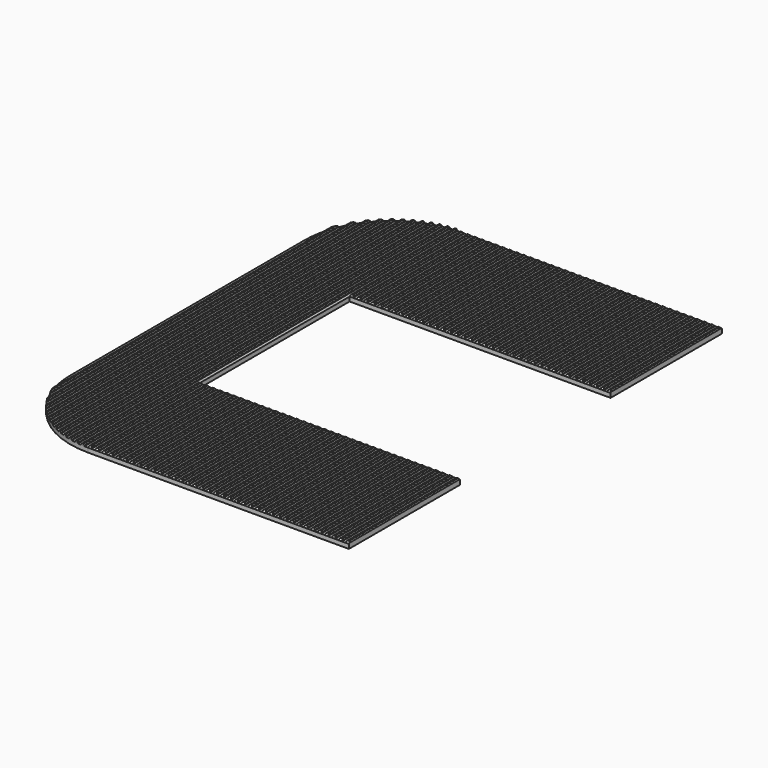
from build123d import *

# Parameters (mm, degrees)
F1_DEPTH = 2.5
F2_R     = 50
F3_W     = 2
F3_H     = 80
F4_DEPTH = 1
F5_SIZE  = 1
F6_SIZE  = 0.6


with BuildPart() as f1:
    # F0 (on Top) → F1 (new body)
    with BuildSketch(Plane.XY):
        Polygon((0, 134), (-200, 134), (-200, -134), (0, -134), (0, -54), (-150, -54), (-150, 54), (0, 54), align=None)
    extrude(amount=F1_DEPTH)

    # F2
    f2_edges = [f1.edges().sort_by_distance(p)[0] for p in [
        (-200, -134, 1.25),
        (-200, 134, 1.25),
    ]]
    fillet(f2_edges, radius=F2_R)

    # F3 (on face) → F4 (join)
    with BuildSketch(Plane.XY.offset(2.5)):
        with BuildLine():
            Line((-196, -103.5959179423), (-196, 103.5959179423))
            ThreePointArc((-196, 103.5959179423), (-197.0832090496, 100.8276981669), (-198, 98))
            Line((-198, 98), (-198, -98))
            ThreePointArc((-198, -98), (-197.0832090496, -100.8276981669), (-196, -103.5959179423))
        make_face()
        with BuildLine():
            Line((-192, -111.1293199325), (-192, 111.1293199325))
            ThreePointArc((-192, 111.1293199325), (-193.0332101351, 109.4586493253), (-194, 107.7486841741))
            Line((-194, 107.7486841741), (-194, -107.7486841741))
            ThreePointArc((-194, -107.7486841741), (-193.0332101351, -109.4586493253), (-192, -111.1293199325))
        make_face()
        with BuildLine():
            Line((-188, -116.4961536185), (-188, 116.4961536185))
            ThreePointArc((-188, 116.4961536185), (-189.0199653475, 115.2640736993), (-190, 114))
            Line((-190, 114), (-190, -114))
            ThreePointArc((-190, -114), (-189.0199653475, -115.2640736993), (-188, -116.4961536185))
        make_face()
        with BuildLine():
            Line((-184, -120.6606055596), (-184, 120.6606055596))
            ThreePointArc((-184, 120.6606055596), (-185.0137439482, 119.6936651905), (-186, 118.6987031458))
            Line((-186, 118.6987031458), (-186, -118.6987031458))
            ThreePointArc((-186, -118.6987031458), (-185.0137439482, -119.6936651905), (-184, -120.6606055596))
        make_face()
        with BuildLine():
            Line((-180, -124), (-180, 124))
            ThreePointArc((-180, 124), (-181.0100804821, 123.2221226923), (-182, 122.4187454246))
            Line((-182, 122.4187454246), (-182, -122.4187454246))
            ThreePointArc((-182, -122.4187454246), (-181.0100804821, -123.2221226923), (-180, -124))
        make_face()
        with BuildLine():
            Line((-176, -126.7083130081), (-176, 126.7083130081))
            ThreePointArc((-176, 126.7083130081), (-177.0076278168, 126.078355953), (-178, 125.4246303544))
            Line((-178, 125.4246303544), (-178, -125.4246303544))
            ThreePointArc((-178, -125.4246303544), (-177.0076278168, -126.078355953), (-176, -126.7083130081))
        make_face()
        with BuildLine():
            Line((-172, -128.8998886413), (-172, 128.8998886413))
            ThreePointArc((-172, 128.8998886413), (-173.0058376186, 128.3929210063), (-174, 127.8634243989))
            Line((-174, 127.8634243989), (-174, -127.8634243989))
            ThreePointArc((-174, -127.8634243989), (-173.0058376186, -128.3929210063), (-172, -128.8998886413))
        make_face()
        with BuildLine():
            Line((-168, -130.6476151588), (-168, 130.6476151588))
            ThreePointArc((-168, 130.6476151588), (-169.0044432365, 130.2474987137), (-170, 129.8257569496))
            Line((-170, 129.8257569496), (-170, -129.8257569496))
            ThreePointArc((-170, -129.8257569496), (-169.0044432365, -130.2474987137), (-168, -130.6476151588))
        make_face()
        with BuildLine():
            Line((-164, -132), (-164, 132))
            ThreePointArc((-164, 132), (-165.003297934, 131.6959227933), (-166, 131.3708771293))
            Line((-166, 131.3708771293), (-166, -131.3708771293))
            ThreePointArc((-166, -131.3708771293), (-165.003297934, -131.6959227933), (-164, -132))
        make_face()
        with BuildLine():
            Line((-160, -132.9897948557), (-160, 132.9897948557))
            ThreePointArc((-160, 132.9897948557), (-161.0023126743, 132.7744719686), (-162, 132.538644398))
            Line((-162, 132.538644398), (-162, -132.538644398))
            ThreePointArc((-162, -132.538644398), (-161.0023126743, -132.7744719686), (-160, -132.9897948557))
        make_face()
        with BuildLine():
            Line((-156, -133.638694584), (-156, 133.638694584))
            ThreePointArc((-156, 133.638694584), (-157.0014284373, 133.5073731866), (-158, 133.355850717))
            Line((-158, 133.355850717), (-158, -133.355850717))
            ThreePointArc((-158, -133.355850717), (-157.0014284373, -133.5073731866), (-156, -133.638694584))
        make_face()
        with BuildLine():
            Line((-152, -133.9599839872), (-152, 133.9599839872))
            ThreePointArc((-152, 133.9599839872), (-153.00060235, 133.909882644), (-154, 133.8397431775))
            Line((-154, 133.8397431775), (-154, -133.8397431775))
            ThreePointArc((-154, -133.8397431775), (-153.00060235, -133.909882644), (-152, -133.9599839872))
        make_face()
        with Locations((-149, -94)):
            Rectangle(F3_W, F3_H)
        with Locations((-145, -94)):
            Rectangle(F3_W, F3_H)
        with Locations((-141, -94)):
            Rectangle(F3_W, F3_H)
        with Locations((-137, -94)):
            Rectangle(F3_W, F3_H)
        with Locations((-133, -94)):
            Rectangle(F3_W, F3_H)
        with Locations((-129, -94)):
            Rectangle(F3_W, F3_H)
        with Locations((-125, -94)):
            Rectangle(F3_W, F3_H)
        with Locations((-121, -94)):
            Rectangle(F3_W, F3_H)
        with Locations((-117, -94)):
            Rectangle(F3_W, F3_H)
        with Locations((-113, -94)):
            Rectangle(F3_W, F3_H)
        with Locations((-109, -94)):
            Rectangle(F3_W, F3_H)
        with Locations((-105, -94)):
            Rectangle(F3_W, F3_H)
        with Locations((-101, -94)):
            Rectangle(F3_W, F3_H)
        with Locations((-97, -94)):
            Rectangle(F3_W, F3_H)
        with Locations((-93, -94)):
            Rectangle(F3_W, F3_H)
        with Locations((-89, -94)):
            Rectangle(F3_W, F3_H)
        with Locations((-85, -94)):
            Rectangle(F3_W, F3_H)
        with Locations((-81, -94)):
            Rectangle(F3_W, F3_H)
        with Locations((-77, -94)):
            Rectangle(F3_W, F3_H)
        with Locations((-73, -94)):
            Rectangle(F3_W, F3_H)
        with Locations((-69, -94)):
            Rectangle(F3_W, F3_H)
        with Locations((-65, -94)):
            Rectangle(F3_W, F3_H)
        with Locations((-61, -94)):
            Rectangle(F3_W, F3_H)
        with Locations((-57, -94)):
            Rectangle(F3_W, F3_H)
        with Locations((-53, -94)):
            Rectangle(F3_W, F3_H)
        with Locations((-49, -94)):
            Rectangle(F3_W, F3_H)
        with Locations((-45, -94)):
            Rectangle(F3_W, F3_H)
        with Locations((-41, -94)):
            Rectangle(F3_W, F3_H)
        with Locations((-37, -94)):
            Rectangle(F3_W, F3_H)
        with Locations((-33, -94)):
            Rectangle(F3_W, F3_H)
        with Locations((-29, -94)):
            Rectangle(F3_W, F3_H)
        with Locations((-25, -94)):
            Rectangle(F3_W, F3_H)
        with Locations((-21, -94)):
            Rectangle(F3_W, F3_H)
        with Locations((-17, -94)):
            Rectangle(F3_W, F3_H)
        with Locations((-13, -94)):
            Rectangle(F3_W, F3_H)
        with Locations((-9, -94)):
            Rectangle(F3_W, F3_H)
        with Locations((-5, -94)):
            Rectangle(F3_W, F3_H)
        with Locations((-1, -94)):
            Rectangle(F3_W, F3_H)
        with Locations((-149, 94)):
            Rectangle(F3_W, F3_H)
        with Locations((-145, 94)):
            Rectangle(F3_W, F3_H)
        with Locations((-141, 94)):
            Rectangle(F3_W, F3_H)
        with Locations((-137, 94)):
            Rectangle(F3_W, F3_H)
        with Locations((-133, 94)):
            Rectangle(F3_W, F3_H)
        with Locations((-129, 94)):
            Rectangle(F3_W, F3_H)
        with Locations((-125, 94)):
            Rectangle(F3_W, F3_H)
        with Locations((-121, 94)):
            Rectangle(F3_W, F3_H)
        with Locations((-117, 94)):
            Rectangle(F3_W, F3_H)
        with Locations((-113, 94)):
            Rectangle(F3_W, F3_H)
        with Locations((-109, 94)):
            Rectangle(F3_W, F3_H)
        with Locations((-105, 94)):
            Rectangle(F3_W, F3_H)
        with Locations((-101, 94)):
            Rectangle(F3_W, F3_H)
        with Locations((-97, 94)):
            Rectangle(F3_W, F3_H)
        with Locations((-93, 94)):
            Rectangle(F3_W, F3_H)
        with Locations((-89, 94)):
            Rectangle(F3_W, F3_H)
        with Locations((-85, 94)):
            Rectangle(F3_W, F3_H)
        with Locations((-81, 94)):
            Rectangle(F3_W, F3_H)
        with Locations((-77, 94)):
            Rectangle(F3_W, F3_H)
        with Locations((-73, 94)):
            Rectangle(F3_W, F3_H)
        with Locations((-69, 94)):
            Rectangle(F3_W, F3_H)
        with Locations((-65, 94)):
            Rectangle(F3_W, F3_H)
        with Locations((-61, 94)):
            Rectangle(F3_W, F3_H)
        with Locations((-57, 94)):
            Rectangle(F3_W, F3_H)
        with Locations((-53, 94)):
            Rectangle(F3_W, F3_H)
        with Locations((-49, 94)):
            Rectangle(F3_W, F3_H)
        with Locations((-45, 94)):
            Rectangle(F3_W, F3_H)
        with Locations((-41, 94)):
            Rectangle(F3_W, F3_H)
        with Locations((-37, 94)):
            Rectangle(F3_W, F3_H)
        with Locations((-33, 94)):
            Rectangle(F3_W, F3_H)
        with Locations((-29, 94)):
            Rectangle(F3_W, F3_H)
        with Locations((-25, 94)):
            Rectangle(F3_W, F3_H)
        with Locations((-21, 94)):
            Rectangle(F3_W, F3_H)
        with Locations((-17, 94)):
            Rectangle(F3_W, F3_H)
        with Locations((-13, 94)):
            Rectangle(F3_W, F3_H)
        with Locations((-9, 94)):
            Rectangle(F3_W, F3_H)
        with Locations((-5, 94)):
            Rectangle(F3_W, F3_H)
        with Locations((-1, 94)):
            Rectangle(F3_W, F3_H)
    extrude(amount=F4_DEPTH)

    # F5
    f5_edges = [f1.edges().sort_by_distance(p)[0] for p in [
        (-5, -54, 3.5),
        (-81, 54, 3.5),
        (-93, -134, 3.5),
        (-85, 134, 3.5),
        (-149, -134, 3.5),
        (-145, -134, 3.5),
        (-141, -134, 3.5),
        (-137, -134, 3.5),
        (-133, -134, 3.5),
        (-129, -134, 3.5),
        (-125, -134, 3.5),
        (-121, -134, 3.5),
        (-117, -134, 3.5),
        (-113, -134, 3.5),
        (-109, -134, 3.5),
        (-105, -134, 3.5),
        (-101, -134, 3.5),
        (-97, -134, 3.5),
        (-89, -134, 3.5),
        (-85, -134, 3.5),
        (-81, -134, 3.5),
        (-77, -134, 3.5),
        (-73, -134, 3.5),
        (-69, -134, 3.5),
        (-65, -134, 3.5),
        (-61, -134, 3.5),
        (-57, -134, 3.5),
        (-53, -134, 3.5),
        (-49, -134, 3.5),
        (-45, -134, 3.5),
        (-41, -134, 3.5),
        (-37, -134, 3.5),
        (-33, -134, 3.5),
        (-29, -134, 3.5),
        (-25, -134, 3.5),
        (-21, -134, 3.5),
        (-17, -134, 3.5),
        (-13, -134, 3.5),
        (-9, -134, 3.5),
        (-5, -134, 3.5),
        (-1, -134, 3.5),
        (-149, 54, 3.5),
        (-145, 54, 3.5),
        (-141, 54, 3.5),
        (-137, 54, 3.5),
        (-133, 54, 3.5),
        (-129, 54, 3.5),
        (-125, 54, 3.5),
        (-121, 54, 3.5),
        (-117, 54, 3.5),
        (-113, 54, 3.5),
        (-109, 54, 3.5),
        (-105, 54, 3.5),
        (-101, 54, 3.5),
        (-97, 54, 3.5),
        (-93, 54, 3.5),
        (-89, 54, 3.5),
        (-85, 54, 3.5),
        (-77, 54, 3.5),
        (-73, 54, 3.5),
        (-69, 54, 3.5),
        (-65, 54, 3.5),
        (-61, 54, 3.5),
        (-57, 54, 3.5),
        (-53, 54, 3.5),
        (-49, 54, 3.5),
        (-45, 54, 3.5),
        (-41, 54, 3.5),
        (-37, 54, 3.5),
        (-33, 54, 3.5),
        (-29, 54, 3.5),
        (-21, 54, 3.5),
        (-25, 54, 3.5),
        (-17, 54, 3.5),
        (-13, 54, 3.5),
        (-9, 54, 3.5),
        (-5, 54, 3.5),
        (-1, 54, 3.5),
        (-1, -54, 3.5),
        (-9, -54, 3.5),
        (-17, -54, 3.5),
        (-21, -54, 3.5),
        (-25, -54, 3.5),
        (-29, -54, 3.5),
        (-33, -54, 3.5),
        (-37, -54, 3.5),
        (-41, -54, 3.5),
        (-45, -54, 3.5),
        (-49, -54, 3.5),
        (-53, -54, 3.5),
        (-57, -54, 3.5),
        (-61, -54, 3.5),
        (-65, -54, 3.5),
        (-69, -54, 3.5),
        (-73, -54, 3.5),
        (-77, -54, 3.5),
        (-81, -54, 3.5),
        (-85, -54, 3.5),
        (-89, -54, 3.5),
        (-93, -54, 3.5),
        (-97, -54, 3.5),
        (-101, -54, 3.5),
        (-105, -54, 3.5),
        (-109, -54, 3.5),
        (-113, -54, 3.5),
        (-117, -54, 3.5),
        (-121, -54, 3.5),
        (-125, -54, 3.5),
        (-129, -54, 3.5),
        (-133, -54, 3.5),
        (-137, -54, 3.5),
        (-141, -54, 3.5),
        (-145, -54, 3.5),
        (-149, -54, 3.5),
        (-13, -54, 3.5),
        (-149, 134, 3.5),
        (-145, 134, 3.5),
        (-141, 134, 3.5),
        (-137, 134, 3.5),
        (-133, 134, 3.5),
        (-129, 134, 3.5),
        (-125, 134, 3.5),
        (-121, 134, 3.5),
        (-117, 134, 3.5),
        (-113, 134, 3.5),
        (-109, 134, 3.5),
        (-105, 134, 3.5),
        (-101, 134, 3.5),
        (-97, 134, 3.5),
        (-93, 134, 3.5),
        (-89, 134, 3.5),
        (-81, 134, 3.5),
        (-77, 134, 3.5),
        (-73, 134, 3.5),
        (-65, 134, 3.5),
        (-61, 134, 3.5),
        (-57, 134, 3.5),
        (-53, 134, 3.5),
        (-49, 134, 3.5),
        (-45, 134, 3.5),
        (-69, 134, 3.5),
        (-41, 134, 3.5),
        (-37, 134, 3.5),
        (-33, 134, 3.5),
        (-29, 134, 3.5),
        (-25, 134, 3.5),
        (-21, 134, 3.5),
        (-17, 134, 3.5),
        (-13, 134, 3.5),
        (-9, 134, 3.5),
        (-5, 134, 3.5),
        (-1, 134, 3.5),
    ]]
    chamfer(f5_edges, length=F5_SIZE)

    # F6
    f6_edges = [f1.edges().sort_by_distance(p)[0] for p in [
        (-148, 94, 3.5),
        (-150, 94, 3.5),
        (-146, 94, 3.5),
        (-144, 94, 3.5),
        (-142, 94, 3.5),
        (-140, 94, 3.5),
        (-138, 94, 3.5),
        (-136, 94, 3.5),
        (-134, 94, 3.5),
        (-132, 94, 3.5),
        (-130, 94, 3.5),
        (-128, 94, 3.5),
        (-126, 94, 3.5),
        (-124, 94, 3.5),
        (-122, 94, 3.5),
        (-120, 94, 3.5),
        (-118, 94, 3.5),
        (-116, 94, 3.5),
        (-114, 94, 3.5),
        (-112, 94, 3.5),
        (-110, 94, 3.5),
        (-108, 94, 3.5),
        (-106, 94, 3.5),
        (-104, 94, 3.5),
        (-100, 94, 3.5),
        (-102, 94, 3.5),
        (-98, 94, 3.5),
        (-96, 94, 3.5),
        (-94, 94, 3.5),
        (-92, 94, 3.5),
        (-90, 94, 3.5),
        (-88, 94, 3.5),
        (-86, 94, 3.5),
        (-84, 94, 3.5),
        (-82, 94, 3.5),
        (-80, 94, 3.5),
        (-78, 94, 3.5),
        (-76, 94, 3.5),
        (-74, 94, 3.5),
        (-72, 94, 3.5),
        (-70, 94, 3.5),
        (-68, 94, 3.5),
        (-66, 94, 3.5),
        (-64, 94, 3.5),
        (-62, 94, 3.5),
        (-60, 94, 3.5),
        (-58, 94, 3.5),
        (-56, 94, 3.5),
        (-54, 94, 3.5),
        (-52, 94, 3.5),
        (-50, 94, 3.5),
        (-48, 94, 3.5),
        (-46, 94, 3.5),
        (-44, 94, 3.5),
        (-42, 94, 3.5),
        (-40, 94, 3.5),
        (-38, 94, 3.5),
        (-36, 94, 3.5),
        (-34, 94, 3.5),
        (-32, 94, 3.5),
        (-30, 94, 3.5),
        (-28, 94, 3.5),
        (-26, 94, 3.5),
        (-24, 94, 3.5),
        (-22, 94, 3.5),
        (-20, 94, 3.5),
        (-18, 94, 3.5),
        (-16, 94, 3.5),
        (-14, 94, 3.5),
        (-12, 94, 3.5),
        (-10, 94, 3.5),
        (-8, 94, 3.5),
        (-6, 94, 3.5),
        (-4, 94, 3.5),
        (-2, 94, 3.5),
        (0, 94, 3.5),
        (-2, -94, 3.5),
        (0, -94, 3.5),
        (-6, -94, 3.5),
        (-4, -94, 3.5),
        (-8, -94, 3.5),
        (-10, -94, 3.5),
        (-12, -94, 3.5),
        (-14, -94, 3.5),
        (-16, -94, 3.5),
        (-18, -94, 3.5),
        (-20, -94, 3.5),
        (-22, -94, 3.5),
        (-26, -94, 3.5),
        (-24, -94, 3.5),
        (-30, -94, 3.5),
        (-28, -94, 3.5),
        (-34, -94, 3.5),
        (-32, -94, 3.5),
        (-38, -94, 3.5),
        (-36, -94, 3.5),
        (-40, -94, 3.5),
        (-42, -94, 3.5),
        (-44, -94, 3.5),
        (-46, -94, 3.5),
        (-48, -94, 3.5),
        (-50, -94, 3.5),
        (-52, -94, 3.5),
        (-54, -94, 3.5),
        (-56, -94, 3.5),
        (-58, -94, 3.5),
        (-60, -94, 3.5),
        (-62, -94, 3.5),
        (-64, -94, 3.5),
        (-66, -94, 3.5),
        (-68, -94, 3.5),
        (-70, -94, 3.5),
        (-72, -94, 3.5),
        (-74, -94, 3.5),
        (-76, -94, 3.5),
        (-78, -94, 3.5),
        (-80, -94, 3.5),
        (-82, -94, 3.5),
        (-84, -94, 3.5),
        (-86, -94, 3.5),
        (-88, -94, 3.5),
        (-90, -94, 3.5),
        (-92, -94, 3.5),
        (-94, -94, 3.5),
        (-96, -94, 3.5),
        (-98, -94, 3.5),
        (-100, -94, 3.5),
        (-102, -94, 3.5),
        (-104, -94, 3.5),
        (-106, -94, 3.5),
        (-108, -94, 3.5),
        (-110, -94, 3.5),
        (-112, -94, 3.5),
        (-114, -94, 3.5),
        (-116, -94, 3.5),
        (-118, -94, 3.5),
        (-120, -94, 3.5),
        (-122, -94, 3.5),
        (-124, -94, 3.5),
        (-126, -94, 3.5),
        (-128, -94, 3.5),
        (-130, -94, 3.5),
        (-132, -94, 3.5),
        (-134, -94, 3.5),
        (-136, -94, 3.5),
        (-138, -94, 3.5),
        (-140, -94, 3.5),
        (-142, -94, 3.5),
        (-144, -94, 3.5),
        (-146, -94, 3.5),
        (-148, -94, 3.5),
        (-150, -94, 3.5),
        (-152, 0, 3.5),
        (-154, 0, 3.5),
        (-156, 0, 3.5),
        (-162, 0, 3.5),
        (-160, 0, 3.5),
        (-164, 0, 3.5),
        (-166, 0, 3.5),
        (-168, 0, 3.5),
        (-170, 0, 3.5),
        (-172, 0, 3.5),
        (-174, 0, 3.5),
        (-176, 0, 3.5),
        (-178, 0, 3.5),
        (-180, 0, 3.5),
        (-182, 0, 3.5),
        (-184, 0, 3.5),
        (-186, 0, 3.5),
        (-188, 0, 3.5),
        (-190, 0, 3.5),
        (-192, 0, 3.5),
        (-194, 0, 3.5),
        (-196, 0, 3.5),
        (-198, 0, 3.5),
        (-158, 0, 3.5),
    ]]
    chamfer(f6_edges, length=F6_SIZE)


solid = f1.part
